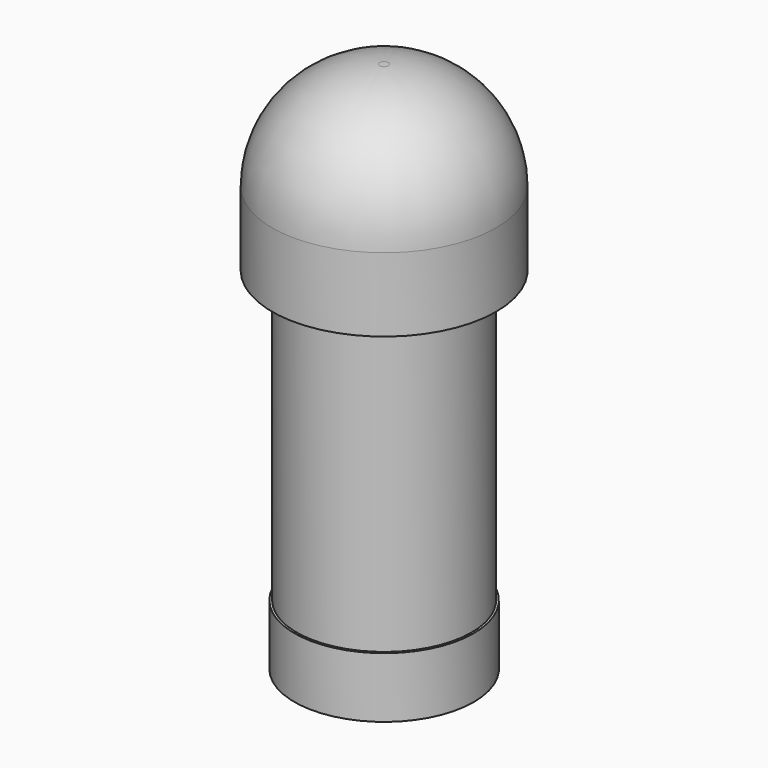
from build123d import *

# Parameters (mm, degrees)
F0_R     = 1.8360694956
F1_DEPTH = 6.096
F2_R     = 2.3520596952
F2_R_2   = 1.8360694956
F3_DEPTH = 3.81
F4_R     = 2.2606
F5_R     = 1.8826071484
F5_R_2   = 1.8360694956
F6_DEPTH = 1.27


with BuildPart() as f1:
    # F0 (on Top) → F1 (new body)
    with BuildSketch(Plane.XY):
        Circle(F0_R)
    extrude(amount=F1_DEPTH)


with BuildPart() as f3:
    # F2 (on face) → F3 (new body)
    with BuildSketch(Plane.XY.offset(6.096)):
        Circle(F2_R)
        Circle(F2_R_2, mode=Mode.SUBTRACT)
        Circle(F2_R_2)
    extrude(amount=F3_DEPTH)

    # F4
    f4_edges = [f3.edges().sort_by_distance(p)[0] for p in [
        (-2.35206, 0, 9.906),
    ]]
    fillet(f4_edges, radius=F4_R)


with BuildPart() as f6:
    # F5 (on face) → F6 (new body)
    with BuildSketch(Plane(origin=(0, 0, 0), x_dir=(1, 0, 0), z_dir=(0, 0, -1))):
        Circle(F5_R)
        Circle(F5_R_2, mode=Mode.SUBTRACT)
        Circle(F5_R_2)
    extrude(amount=F6_DEPTH)


solid = Compound([f1.part, f3.part, f6.part])
